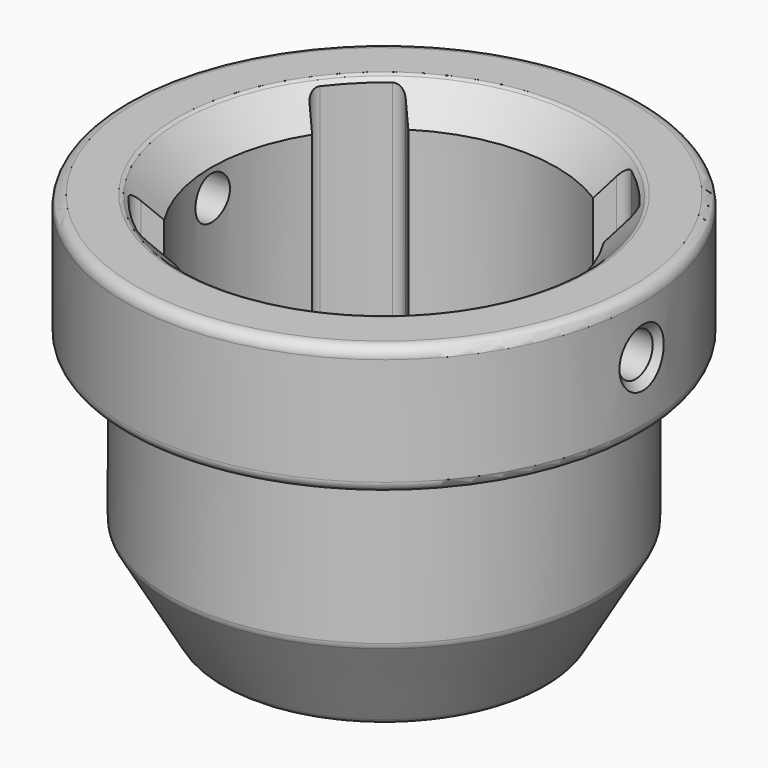
from build123d import *

# Parameters (mm, degrees)
F3_DEPTH = 50
F4_R     = 1
F7_R     = 1
F8_R     = 1
F9_R     = 0.5


with BuildPart() as f1:
    # F0 (on Front) → F1 (revolve)
    with BuildSketch(Plane.XZ):
        with BuildLine():
            Line((-6.5, 0), (-6, 0.5))
            Line((-6, 0.5), (-6, 13))
            Line((-6, 13), (-8, 13))
            Line((-8, 13), (-9, 12))
            Line((-9, 12), (-9, 2.5))
            Line((-9, 2.5), (-14, 2.5))
            Line((-14, 2.5), (-14, 16))
            Line((-14, 16), (-16, 16))
            Line((-16, 16), (-16, 33))
            Line((-16, 33), (-19, 36))
            Line((-19, 36), (-23, 36))
            ThreePointArc((-23, 36), (-23.7071067812, 35.7071067812), (-24, 35))
            Line((-24, 35), (-24, 25))
            ThreePointArc((-24, 25), (-23.7071067812, 24.2928932188), (-23, 24))
            Line((-23, 24), (-21, 24))
            ThreePointArc((-21, 24), (-20.2928932188, 23.7071067812), (-20, 23))
            Line((-20, 23), (-20, 9.5))
            Line((-20, 9.5), (-14.8038475773, 0.5))
            Line((-14.8038475773, 0.5), (-8, 0.5))
            Line((-8, 0.5), (-8, 0))
            Line((-8, 0), (-6.5, 0))
        make_face()
    revolve(axis=Axis((0, 0, 30), (0, 0, 1)))

    # F2 (on face) → F3 (cut)
    with BuildSketch(Plane.XY.offset(16)):
        with BuildLine():
            Line((7.1102710222, -12.0600184905), (10.3703588445, -15.3201063128))
            ThreePointArc((10.3703588445, -15.3201063128), (13.081475452, -13.081475452), (15.3201063128, -10.3703588445))
            Line((15.3201063128, -10.3703588445), (12.0600184905, -7.1102710222))
            ThreePointArc((12.0600184905, -7.1102710222), (14, 0), (12.0600184905, 7.1102710222))
            Line((12.0600184905, 7.1102710222), (15.3201063128, 10.3703588445))
            ThreePointArc((15.3201063128, 10.3703588445), (13.081475452, 13.081475452), (10.3703588445, 15.3201063128))
            Line((10.3703588445, 15.3201063128), (7.1102710222, 12.0600184905))
            ThreePointArc((7.1102710222, 12.0600184905), (0, 14), (-7.1102710222, 12.0600184905))
            Line((-7.1102710222, 12.0600184905), (-10.3703588445, 15.3201063128))
            ThreePointArc((-10.3703588445, 15.3201063128), (-13.081475452, 13.081475452), (-15.3201063128, 10.3703588445))
            Line((-15.3201063128, 10.3703588445), (-12.0600184905, 7.1102710222))
            ThreePointArc((-12.0600184905, 7.1102710222), (-14, 0), (-12.0600184905, -7.1102710222))
            Line((-12.0600184905, -7.1102710222), (-15.3201063128, -10.3703588445))
            ThreePointArc((-15.3201063128, -10.3703588445), (-13.081475452, -13.081475452), (-10.3703588445, -15.3201063128))
            Line((-10.3703588445, -15.3201063128), (-7.1102710222, -12.0600184905))
            ThreePointArc((-7.1102710222, -12.0600184905), (-5.3575680531, -12.9343134552), (-3.5, -13.5554417117))
            Line((-3.5, -13.5554417117), (-3.5, -18.1659021246))
            ThreePointArc((-3.5, -18.1659021246), (0, -18.5), (3.5, -18.1659021246))
            Line((3.5, -18.1659021246), (3.5, -13.5554417117))
            ThreePointArc((3.5, -13.5554417117), (5.3575680531, -12.9343134552), (7.1102710222, -12.0600184905))
        make_face()
    extrude(amount=F3_DEPTH, mode=Mode.SUBTRACT)

    # F4
    f4_edges = [f1.edges().sort_by_distance(p)[0] for p in [
        (-10.370359, 15.320106, 25.75),
        (10.370359, 15.320106, 25.75),
        (10.370359, -15.320106, 25.75),
        (-10.370359, -15.320106, 25.75),
        (3.5, -18.165902, 25.75),
        (15.320106, 10.370359, 25.75),
        (15.320106, -10.370359, 25.75),
        (-15.320106, 10.370359, 25.75),
        (-3.5, -18.165902, 25.75),
        (-15.320106, -10.370359, 25.75),
    ]]
    fillet(f4_edges, radius=F4_R)

    # F5 (on Front) → F6 (revolve, cut)
    with BuildSketch(Plane.XZ):
        Polygon((24, 30.5), (-24, 30.5), (-24, 27.8), (-23.3, 28.5), (23.3, 28.5), (24, 27.8), align=None)
    revolve(axis=Axis((0, 0, 30.5), (-1, 0, 0)), mode=Mode.SUBTRACT)

    # F7
    f7_edges = [f1.edges().sort_by_distance(p)[0] for p in [
        (14, 0, 2.5),
        (9, 0, 2.5),
    ]]
    fillet(f7_edges, radius=F7_R)

    # F8
    f8_edges = [f1.edges().sort_by_distance(p)[0] for p in [
        (20, 0, 9.5),
        (14.803848, 0, 0.5),
    ]]
    fillet(f8_edges, radius=F8_R)

    # F9
    f9_edges = [f1.edges().sort_by_distance(p)[0] for p in [
        (19, 0, 36),
    ]]
    fillet(f9_edges, radius=F9_R)


solid = f1.part
